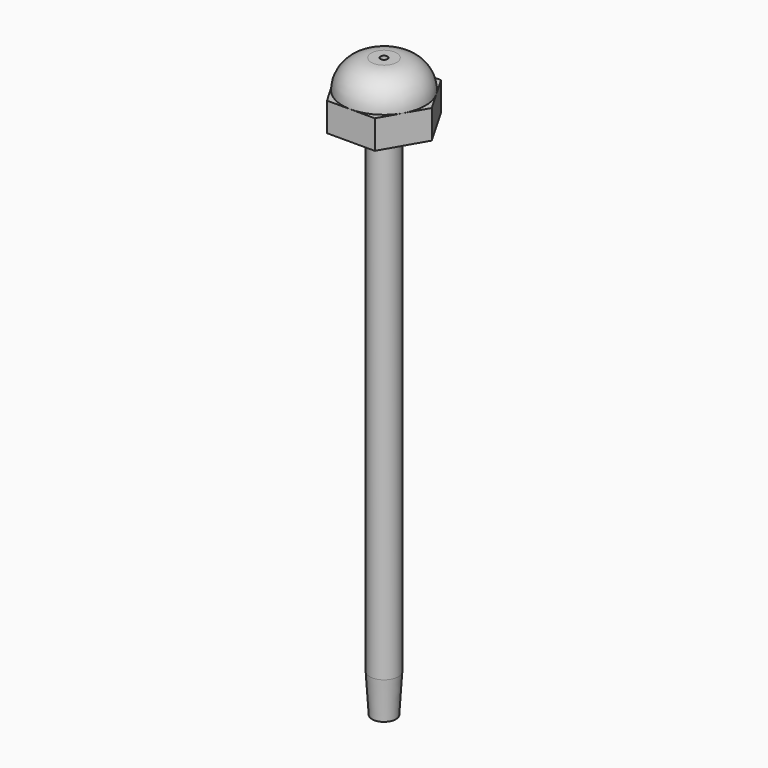
from build123d import *

# Parameters (mm, degrees)
F0_R     = 3
F1_DEPTH = 6
F2_R     = 8.6602540378
F3_DEPTH = 6
F4_R     = 5.99999
F5_R     = 0.75
F6_DEPTH = 3
F7_R     = 3
F8_DEPTH = 101
F10_R    = 2.5
F11_R    = 3


# Not quite as in the source:
# - a fillet or chamfer is up to 0.001 mm smaller than in the source, because OpenCascade refuses the exact size


with BuildPart() as f1:
    # F0 (on Top) → F1 (new body)
    with BuildSketch(Plane.XY):
        Polygon((5, 8.6602540378), (-5, 8.6602540378), (-10, 0), (-5, -8.6602540378), (5, -8.6602540378), (10, 0), align=None)
        Circle(F0_R, mode=Mode.SUBTRACT)
        Circle(F0_R)
    extrude(amount=F1_DEPTH)

    # F2 (on face) → F3 (join)
    with BuildSketch(Plane.XY.offset(6)):
        Circle(F2_R)
    extrude(amount=F3_DEPTH)

    # F4 (radius 6 in the source; OpenCascade refuses exactly that, so slightly less here)
    f4_edges = [f1.edges().sort_by_distance(p)[0] for p in [
        (-8.660254, 0, 12),
    ]]
    fillet(f4_edges, radius=F4_R)

    # F5 (on face) → F6 (cut)
    with BuildSketch(Plane.XY.offset(12)):
        Circle(F5_R)
    extrude(amount=-F6_DEPTH, mode=Mode.SUBTRACT)

    # F7 (on face) → F8 (join)
    with BuildSketch(Plane(origin=(0, 0, 0), x_dir=(1, 0, 0), z_dir=(0, 0, -1))):
        Circle(F7_R)
    extrude(amount=F8_DEPTH)

    # F10 (on offset) → F12 section 0
    with BuildSketch(Plane(origin=(0, 0, -109), x_dir=(1, 0, 0), z_dir=(0, 0, -1))):
        Circle(F10_R)
    # F11 (on face) → F12 section 1
    with BuildSketch(Plane(origin=(0, 0, -101), x_dir=(1, 0, 0), z_dir=(0, 0, -1))):
        Circle(F11_R)
    loft()


solid = f1.part
